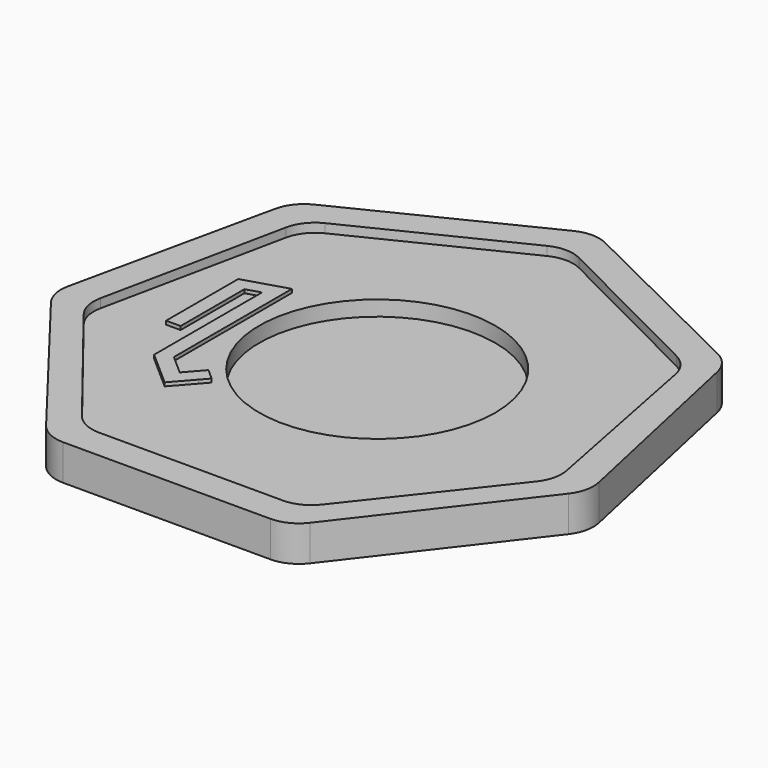
from build123d import *

# Parameters (mm, degrees)
F0_R     = 6.6066656701
F1_DEPTH = 1.5
F2_DEPTH = 2
F3_DEPTH = 0.65
F5_DEPTH = 1.7


# Not quite as in the source:
# - a feature names something its author has since deleted; it is built from what else it names


with BuildPart() as f1:
    # F0 (on Top) → F1 (new body)
    with BuildSketch(Plane.XY):
        with BuildLine():
            ThreePointArc((0.8885468305, 16.9870886264), (-0.0010928636, 17.2005022258), (-0.8926896019, 16.9954183263))
            Line((-0.8926896019, 16.9954183263), (-9.8272421593, 12.6038188933))
            ThreePointArc((-9.8272421593, 12.6038188933), (-10.5252186518, 12.034854024), (-10.9028479986, 11.2173650131))
            Line((-10.9028479986, 11.2173650131), (-13.052575898, 0.9126909889))
            ThreePointArc((-13.052575898, 0.9126909889), (-13.0418066326, 0.0472202699), (-12.6663707931, -0.732653741))
            Line((-12.6663707931, -0.732653741), (-6.7182242373, -8.2905330076))
            ThreePointArc((-6.7182242373, -8.2905330076), (-6.0201328246, -8.8527685293), (-5.146579379, -9.0536286299))
            Line((-5.146579379, -9.0536286299), (5.146579379, -9.0536286299))
            ThreePointArc((5.146579379, -9.0536286299), (6.0201328246, -8.8527685293), (6.7182242373, -8.2905330076))
            Line((6.7182242373, -8.2905330076), (12.6752768476, -0.7213374622))
            ThreePointArc((12.6752768476, -0.7213374622), (13.0479677297, 0.0469961856), (13.0661891506, 0.9007543878))
            Line((13.0661891506, 0.9007543878), (11.0860832533, 10.9895326776))
            ThreePointArc((11.0860832533, 10.9895326776), (10.7166616036, 11.8134437296), (10.0225184006, 12.3909097378))
            Line((10.0225184006, 12.3909097378), (0.8885468305, 16.9870886264))
        make_face()
        with Locations((0, 3.9848611549)):
            Circle(F0_R, mode=Mode.SUBTRACT)
    extrude(amount=F1_DEPTH)

    # F0 (on Top) → F2 (join)
    with BuildSketch(Plane.XY):
        with BuildLine():
            Line((-5.7990739843, -10.7466970864), (5.7990739843, -10.7466970864))
            ThreePointArc((5.7990739843, -10.7466970864), (6.6819267685, -10.541292016), (7.3834371144, -9.9672680479))
            Line((7.3834371144, -9.9672680479), (14.4937978518, -0.737658505))
            ThreePointArc((14.4937978518, -0.737658505), (14.8609319824, 0.0451243323), (14.8633622841, 0.9097228137))
            Line((14.8633622841, 0.9097228137), (12.3725781296, 12.3124728375))
            ThreePointArc((12.3725781296, 12.3124728375), (11.9938877885, 13.1179886127), (11.3031972843, 13.6794230844))
            Line((11.3031972843, 13.6794230844), (0.8845467171, 18.817111544))
            ThreePointArc((0.8845467171, 18.817111544), (0, 19.0233509398), (-0.8845467171, 18.817111544))
            Line((-0.8845467171, 18.817111544), (-11.3031972843, 13.6794230844))
            ThreePointArc((-11.3031972843, 13.6794230844), (-11.9938877885, 13.1179886127), (-12.3725781296, 12.3124728375))
            Line((-12.3725781296, 12.3124728375), (-14.8633622841, 0.9097228137))
            ThreePointArc((-14.8633622841, 0.9097228137), (-14.8609319824, 0.0451243323), (-14.4937978518, -0.737658505))
            Line((-14.4937978518, -0.737658505), (-7.3834371144, -9.9672680479))
            ThreePointArc((-7.3834371144, -9.9672680479), (-6.6819267685, -10.541292016), (-5.7990739843, -10.7466970864))
        make_face()
        with BuildLine():
            Line((-9.8272421593, 12.6038188933), (-0.8926896019, 16.9954183263))
            ThreePointArc((-0.8926896019, 16.9954183263), (-0.0010928636, 17.2005022258), (0.8885468305, 16.9870886264))
            Line((0.8885468305, 16.9870886264), (10.0225184006, 12.3909097378))
            ThreePointArc((10.0225184006, 12.3909097378), (10.7166616036, 11.8134437296), (11.0860832533, 10.9895326776))
            Line((11.0860832533, 10.9895326776), (13.0661891506, 0.9007543878))
            ThreePointArc((13.0661891506, 0.9007543878), (13.0479677297, 0.0469961856), (12.6752768476, -0.7213374622))
            Line((12.6752768476, -0.7213374622), (6.7182242373, -8.2905330076))
            ThreePointArc((6.7182242373, -8.2905330076), (6.0201328246, -8.8527685293), (5.146579379, -9.0536286299))
            Line((5.146579379, -9.0536286299), (-5.146579379, -9.0536286299))
            ThreePointArc((-5.146579379, -9.0536286299), (-6.0201328246, -8.8527685293), (-6.7182242373, -8.2905330076))
            Line((-6.7182242373, -8.2905330076), (-12.6663707931, -0.732653741))
            ThreePointArc((-12.6663707931, -0.732653741), (-13.0418066326, 0.0472202699), (-13.052575898, 0.9126909889))
            Line((-13.052575898, 0.9126909889), (-10.9028479986, 11.2173650131))
            ThreePointArc((-10.9028479986, 11.2173650131), (-10.5252186518, 12.034854024), (-9.8272421593, 12.6038188933))
        make_face(mode=Mode.SUBTRACT)
    extrude(amount=F2_DEPTH)

    # F0 (on Top) → F3 (join)
    with BuildSketch(Plane.XY):
        with Locations((0, 3.9848611549)):
            Circle(F0_R)
    extrude(amount=F3_DEPTH)

    # F4 (on Top) → F5 (join)
    with BuildSketch(Plane.XY):
        Polygon((-6.2406868358, -3.0968557074), (-5.2452536218, -1.9672723198), (-4.8604047071, -1.5305590028), (-5.0104551537, -1.3983286602), (-5.3199341997, -1.1256035787), (-5.4699846462, -0.9933732362), (-5.8548335609, -1.4300865532), (-6.3130810083, -1.9500900017), (-7.3554360868, -1.0315257971), (-7.4232057442, -0.9718045152), (-7.4232057442, -0.8814753506), (-7.4232057442, 7.291526825), (-9.6988570439, 6.5962814227), (-9.8404204473, 6.5530316922), (-9.8404204473, 6.405008936), (-9.8404204473, 1.7031954848), (-9.8404204473, 1.5031954848), (-9.6404204473, 1.5031954848), (-9.2274204473, 1.5031954848), (-9.0274204473, 1.5031954848), (-9.0274204473, 1.7031954848), (-9.0274204473, 5.8236241114), (-9.0274204473, 5.9716468677), (-8.8858570439, 6.0148965982), (-8.2362057442, 6.2133747566), (-8.2362057442, -0.8866803037), (-8.2362057442, -1.3383261269), (-7.897357457, -1.6369325365), align=None)
    extrude(amount=F5_DEPTH)


solid = f1.part
